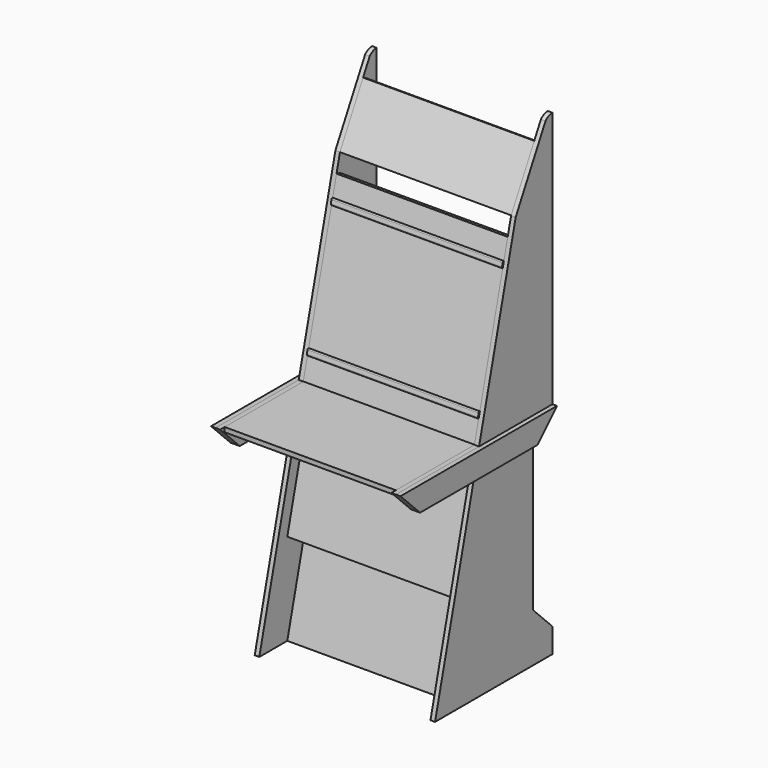
from build123d import *

# Parameters (mm, degrees)
F1_DEPTH  = 19.05
F3_DEPTH  = 25.4
F6_DEPTH  = 19.05
F9_DEPTH  = 711.2
F11_W     = 711.2
F11_H     = 508
F12_DEPTH = 19.05
F13_DEPTH = 19.05
F15_W     = 311.15
F15_H     = 431.8
F16_DEPTH = 44.45
F18_DEPTH = 19.05
F19_W     = 711.2
F19_H     = 101.6
F20_DEPTH = 19.05
F21_W     = 711.2
F21_H     = 508
F22_DEPTH = 5.08
F23_W     = 711.2
F23_H     = 254
F24_DEPTH = 19.05
F25_W     = 711.2
F25_H     = 12.7
F26_DEPTH = 5.08
F27_R     = 5.07999
F30_DEPTH = 762


# Not quite as in the source:
# - a fillet or chamfer is up to 0.001 mm smaller than in the source, because OpenCascade refuses the exact size


with BuildPart() as f1:
    # F0 (on Right) → F1 (new body)
    with BuildSketch(Plane.YZ):
        Polygon((-609.6, -978.4476216069), (0, -978.4476216069), (0, 1053.5523783931), (-190.5, 697.9523783931), align=None)
    extrude(amount=F1_DEPTH)

    # F2 (on face) → F3 (cut)
    with BuildSketch(Plane.YZ.offset(19.05)):
        Polygon((-101.599991038, -775.2476216069), (0, -876.8476216069), (0, -64.0476216069), (-101.599991038, -165.6476216069), align=None)
    extrude(amount=-F3_DEPTH, mode=Mode.SUBTRACT)


with BuildPart() as f4_1:
    # F4: copy of F1
    add(f1.part.moved(Location((730.25, 0, 0))))


with BuildPart() as f6:
    # F5 (on face) → F6 (new body)
    with BuildSketch(Plane.YZ.offset(749.3)):
        Polygon((-101.599991038, -165.6476216069), (8.962e-06, -64.047630569), (-381.0000022405, -64.047630569), (-406.4, -165.6476216069), align=None)
        Polygon((-406.4, -165.6476216069), (-381.0000022405, -64.047630569), (-812.799991038, -64.047630569), (-711.199991038, -165.6476216069), align=None)
    extrude(amount=F6_DEPTH)


with BuildPart() as f7_1:
    # F7: copy of F6
    add(f6.part.moved(Location((-768.35, 0, 0))))


with BuildPart() as f9:
    # F8 (on face) → F9 (new body)
    with BuildSketch(Plane.YZ.offset(19.05)):
        Polygon((-341.0134917488, -485.6152315331), (-464.2215892673, -978.4476216069), (-445.1715892673, -978.4476216069), (-321.9634917488, -485.6152315331), align=None)
    extrude(amount=F9_DEPTH)


with BuildPart() as f10_1:
    # F10: copy of F9
    add(f9.part.moved(Location((0, 0, 381))))


with BuildPart() as f12:
    # F11 (on face) → F12 (new body)
    with BuildSketch(Plane.XY.offset(-64.047630569)):
        with Locations((374.65, -535.5325455644)):
            Rectangle(F11_W, F11_H)
    extrude(amount=-F12_DEPTH)


with BuildPart() as f13:
    # F5 (on face) → F13 (new body)
    with BuildSketch(Plane.YZ.offset(749.3)):
        Polygon((-406.4, -165.6476216069), (-381.0000022405, -64.047630569), (-812.799991038, -64.047630569), (-711.199991038, -165.6476216069), align=None)
    extrude(amount=-F13_DEPTH)


with BuildPart() as f14_1:
    # F14: copy of F13
    add(f13.part.moved(Location((-730.25, 0, 0))))


with BuildPart() as f16:
    # F15 (on face) → F16 (new body)
    with BuildSketch(Plane(origin=(0, -343.5182066807, 85.8795516702), x_dir=(1, 0, 0), z_dir=(0, -0.9701425001, 0.242535625))):
        with Locations((219.075, 250.5829996449)):
            Rectangle(F15_W, F15_H)
        with Locations((530.225, 250.5829996449)):
            Rectangle(F15_W, F15_H)
    extrude(amount=-F16_DEPTH)


with BuildPart() as f18:
    # F17 (on face) → F18 (new body)
    with BuildSketch(Plane(origin=(0, -343.5182066807, 85.8795516702), x_dir=(1, 0, 0), z_dir=(0, -0.9701425001, 0.242535625))):
        Polygon((730.25, -52.3646834135), (19.05, -52.3646834135), (19.05, -153.9646834135), (730.8220367045, -153.9646834135), align=None)
    extrude(amount=-F18_DEPTH)


with BuildPart() as f20:
    # F19 (on face) → F20 (new body)
    with BuildSketch(Plane(origin=(0, -343.5182066807, 85.8795516702), x_dir=(1, 0, 0), z_dir=(0, -0.9701425001, 0.242535625))):
        with Locations((374.65, 506.4353165865)):
            Rectangle(F19_W, F19_H)
    extrude(amount=-F20_DEPTH)


with BuildPart() as f22:
    # F21 (on face) → F22 (new body)
    with BuildSketch(Plane(origin=(0, -343.5182066807, 85.8795516702), x_dir=(1, 0, 0), z_dir=(0, -0.9701425001, 0.242535625))):
        with Locations((374.65, 201.6353165865)):
            Rectangle(F21_W, F21_H)
    extrude(amount=-F22_DEPTH)


with BuildPart() as f24:
    # F23 (on face) → F24 (new body)
    with BuildSketch(Plane(origin=(0, -438.5450930873, 234.9348712968), x_dir=(1, 0, 0), z_dir=(0, -0.88147997, 0.4722214125))):
        with Locations((374.65, 652.2728625032)):
            Rectangle(F23_W, F23_H)
    extrude(amount=-F24_DEPTH)


with BuildPart() as f26:
    # F25 (on face) → F26 (new body)
    with BuildSketch(Plane(origin=(0, -343.5182066807, 85.8795516702), x_dir=(1, 0, 0), z_dir=(0, -0.9701425001, 0.242535625))):
        with Locations((374.7215045881, -46.0146834135)):
            Rectangle(F25_W, F25_H)
        with Locations((374.7215045881, -58.7146834135)):
            Rectangle(F25_W, F25_H)
    extrude(amount=F26_DEPTH)

    # F27 (radius 5.08 in the source; OpenCascade refuses exactly that, so slightly less here)
    f27_edges = [f26.edges().sort_by_distance(p)[0] for p in [
        (374.721505, -358.066629, 48.631238),
        (374.721505, -364.227034, 23.989618),
    ]]
    fillet(f27_edges, radius=F27_R)


with BuildPart() as f28_1:
    # F28: copy of F26
    add(f26.part.moved(Location((0, 124.714, 499.364))))


with BuildPart() as f30_tool:
    # F29 (on face) → F30 (new body)
    with BuildSketch(Plane.YZ.offset(749.3)):
        with BuildLine():
            Line((0, 1053.5523783931), (-35.9832716337, 986.3836046769))
            ThreePointArc((-35.9832716337, 986.3836046769), (-19.6541881516, 998.0758132072), (0, 1002.2061395602))
            Line((0, 1002.2061395602), (0, 1053.5523783931))
        make_face()
    extrude(amount=-F30_DEPTH)


with BuildPart() as f1_1:
    add(f1.part)

    # F30: cut by f30_tool
    add(f30_tool.part, mode=Mode.SUBTRACT)


with BuildPart() as f4_1_1:
    add(f4_1.part)

    # F30: cut by f30_tool
    add(f30_tool.part, mode=Mode.SUBTRACT)


solid = Compound([f6.part, f7_1.part, f9.part, f10_1.part, f12.part, f13.part, f14_1.part, f16.part, f18.part, f20.part, f22.part, f24.part, f26.part, f28_1.part, f1_1.part, f4_1_1.part])
